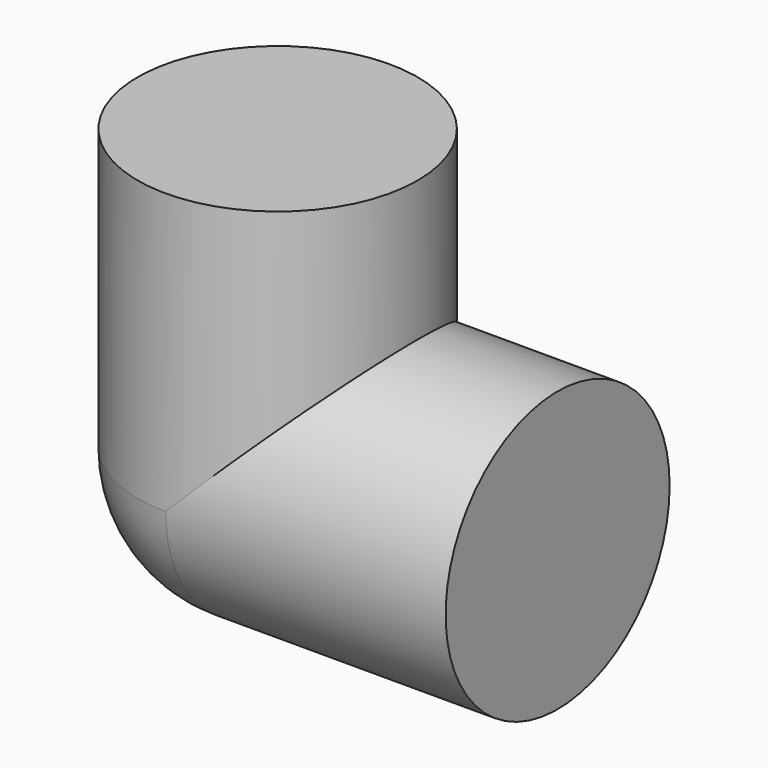
from build123d import *

# Parameters (mm, degrees)
F2_R     = 12.7
F3_DEPTH = 25.4
F7_R     = 12.7
F8_DEPTH = 25.4


# Not quite as in the source:
# - the program builds the solid bodies; features that only make, move or delete a surface that nothing else refers to are left out


with BuildPart() as f1:
    # F0 (on Front) → F1 (revolve)
    with BuildSketch(Plane.XZ):
        with BuildLine():
            ThreePointArc((0, -12.7), (8.9802561211, -8.9802561211), (12.7, 0))
            ThreePointArc((12.7, 0), (8.9802561211, 8.9802561211), (0, 12.7))
            Line((0, 12.7), (0, -12.7))
        make_face()
    revolve(axis=Axis((0, 0, -1.3322243467), (0, 0, -1)))

    # F2 (on Right) → F3 (join)
    with BuildSketch(Plane.YZ):
        Circle(F2_R)
    extrude(amount=F3_DEPTH)

    # F7 (on Top) → F8 (join)
    with BuildSketch(Plane.XY):
        Circle(F7_R)
    extrude(amount=F8_DEPTH)


solid = f1.part
